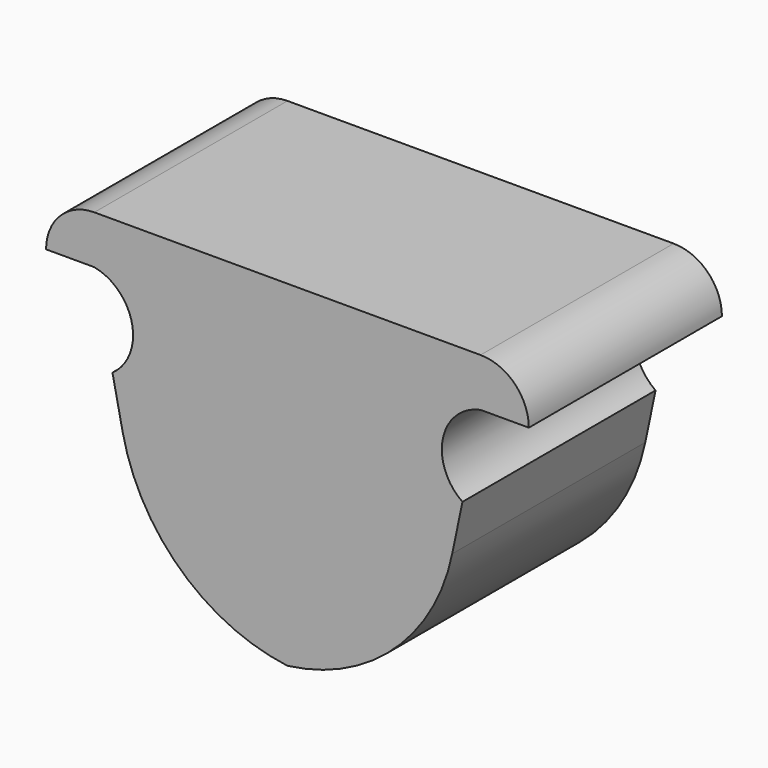
from build123d import *

# Parameters (mm, degrees)
F1_DEPTH    = 5
F2_T1_DEPTH = 21.2627511202


# Not quite as in the source:
# - a fillet or chamfer that OpenCascade refuses, or shapes differently, is made with other operations: its cross-section is extruded or revolved along the edge and cut away or added


with BuildPart() as f1:
    # F0 (on Front) → F1 (new body)
    with BuildSketch(Plane.XZ):
        with BuildLine():
            Line((4, -0.5), (5, -0.5))
            ThreePointArc((5, -0.5), (4.7071067812, 0.2071067812), (4, 0.5))
            Line((4, 0.5), (-4, 0.5))
            ThreePointArc((-4, 0.5), (-4.7071067812, 0.2071067812), (-5, -0.5))
            Line((-5, -0.5), (-4, -0.5))
            ThreePointArc((-4, -0.5), (-3.2187502413, -1.2763021336), (-3.625, -2.3))
            Line((-3.625, -2.3), (-2.75, -6.5))
            Line((-2.75, -6.5), (0, -6.5))
            Line((0, -6.5), (2.75, -6.5))
            Line((2.75, -6.5), (3.625, -2.3))
            ThreePointArc((3.625, -2.3), (3.2187502413, -1.2763021336), (4, -0.5))
        make_face()
    extrude(amount=F1_DEPTH)

    # F2: fillet of radius 4 on 2 edges, made by hand

    # F2_s2 → F2_t1 (cut)
    with BuildSketch(Plane.XZ.offset(-8.1313755601)):
        with BuildLine():
            ThreePointArc((0.502550224, -6.5), (-2.0210119343, -5.6034873985), (-3.4133714549, -3.3158170164))
            Line((-3.4133714549, -3.3158170164), (-2.75, -6.5))
            Line((-2.75, -6.5), (0.502550224, -6.5))
        make_face()
        with BuildLine():
            ThreePointArc((3.4133714549, -3.3158170164), (2.0210119343, -5.6034873985), (-0.502550224, -6.5))
            Line((-0.502550224, -6.5), (2.75, -6.5))
            Line((2.75, -6.5), (3.4133714549, -3.3158170164))
        make_face()
    extrude(amount=F2_T1_DEPTH, mode=Mode.SUBTRACT)


solid = f1.part
